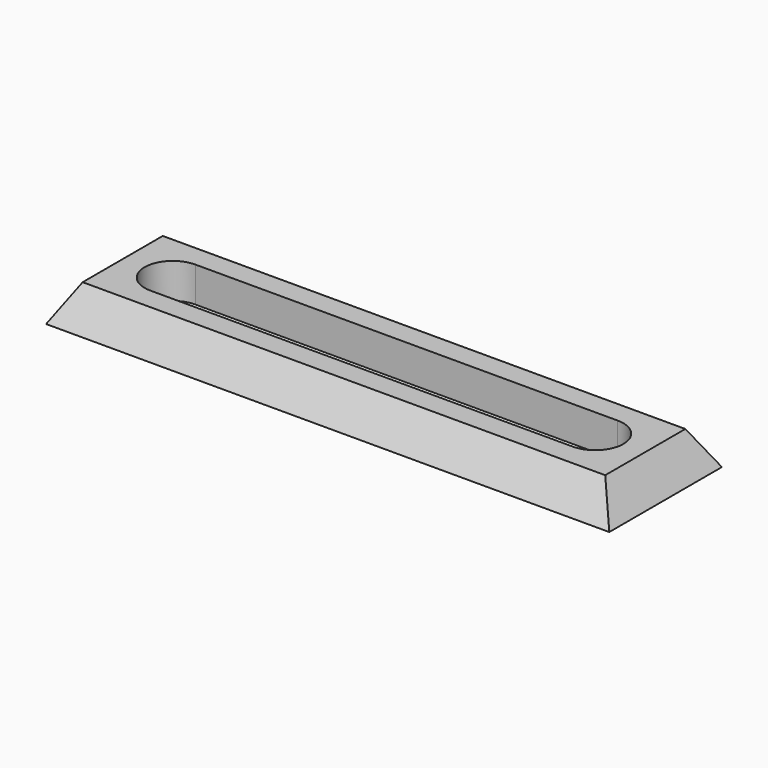
from build123d import *

# Parameters (mm, degrees)
F0_W     = 101.6
F0_H     = 25.4
F1_DEPTH = 6.35
F2_SIZE2 = 3.666164
F2_SIZE  = 6.34999
F4_DEPTH = 42.2284360975


# Not quite as in the source:
# - a fillet or chamfer is up to 0.001 mm smaller than in the source, because OpenCascade refuses the exact size


with BuildPart() as f1:
    # F0 (on Top) → F1 (new body)
    with BuildSketch(Plane.XY):
        Rectangle(F0_W, F0_H)
    extrude(amount=F1_DEPTH)

    # F2 (size 6.35 and 3.6661742094 in the source; OpenCascade refuses exactly that, so slightly less here)
    f2_edges = [f1.edges().sort_by_distance(p)[0] for p in [
        (0, 12.7, 6.35),
        (-50.8, 0, 6.35),
        (0, -12.7, 6.35),
        (50.8, 0, 6.35),
    ]]
    chamfer(f2_edges, length=F2_SIZE, length2=F2_SIZE2)

    # F3 (on face) → F4 (cut)
    with BuildSketch(Plane.XY):
        with BuildLine():
            ThreePointArc((-38.1, 5.08), (-43.18, 0), (-38.1, -5.08))
            Line((-38.1, -5.08), (38.1, -5.08))
            ThreePointArc((38.1, -5.08), (43.18, 0), (38.1, 5.08))
            Line((38.1, 5.08), (-38.1, 5.08))
        make_face()
    extrude(amount=F4_DEPTH, mode=Mode.SUBTRACT)


solid = f1.part
